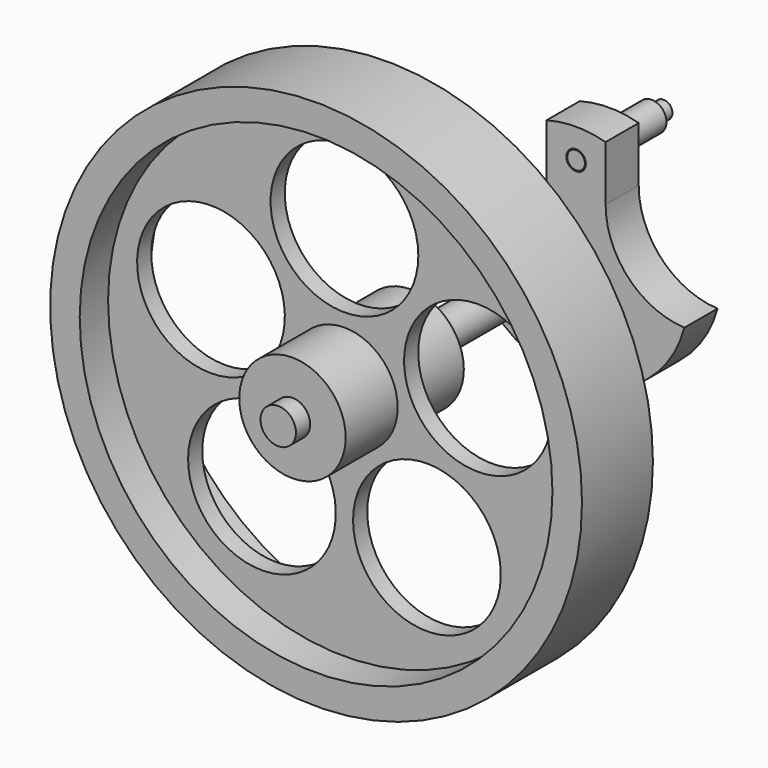
from build123d import *

# Parameters (mm, degrees)
F1_DEPTH         = 7
F2_D             = 6
F3_D             = 3.3
F4_R             = 2.5
F5_DEPTH         = 9
F6_R             = 2
F7_DEPTH         = 7
F8_R             = 1.5
F9_DEPTH         = 3
F10_SIZE         = 0.5
F11_R            = 3
F12_DEPTH        = 70
F16_D            = 6
F17_R            = 12.5
F18_DEPTH        = 68.001
F18_COPIES_COUNT = 5


# Not quite as in the source:
# - a pattern or mirror of a feature is missing from the dataset's text; its kind, count and spacing are read off the source's solid


with BuildPart() as f1:
    # F0 (on Front) → F1 (new body)
    with BuildSketch(Plane.XZ):
        with BuildLine():
            Line((5, 9), (5, 18.3303027798))
            ThreePointArc((5, 18.3303027798), (0, 19), (-5, 18.3303027798))
            Line((-5, 18.3303027798), (-5, 9))
            ThreePointArc((-5, 9), (-8.8679852531, -0.6613807072), (-18.3346110241, -4.9841788286))
            ThreePointArc((-18.3346110241, -4.9841788286), (0, -19), (18.3346110241, -4.9841788286))
            ThreePointArc((18.3346110241, -4.9841788286), (8.8679852531, -0.6613807072), (5, 9))
        make_face()
    extrude(amount=F1_DEPTH)

    # F2 (through all)
    with Locations(Plane(origin=(0, 0, 0), x_dir=(1, 0, 0), z_dir=(0, 1, 0))):
        with Locations((0, 0)):
            Hole(F2_D / 2)

    # F3 (through all)
    with Locations(Plane(origin=(0, 0, 0), x_dir=(1, 0, 0), z_dir=(0, 1, 0))):
        with Locations((0, -14)):
            Hole(F3_D / 2)


with BuildPart() as f5:
    # F4 (on face) → F5 (new body)
    with BuildSketch(Plane(origin=(0, 0, 0), x_dir=(-1, 0, 0), z_dir=(0, 1, 0))):
        with Locations((0, 14)):
            Circle(F4_R)
    extrude(amount=F5_DEPTH)

    # F6 (on face) → F7 (join)
    with BuildSketch(Plane.XZ):
        with Locations((0, 14)):
            Circle(F6_R)
    extrude(amount=F7_DEPTH)

    # F8 (on face) → F9 (join)
    with BuildSketch(Plane(origin=(0, 9, 0), x_dir=(-1, 0, 0), z_dir=(0, 1, 0))):
        with Locations((0, 14)):
            Circle(F8_R)
    extrude(amount=F9_DEPTH)

    # F10
    f10_edges = [f5.edges().sort_by_distance(p)[0] for p in [
        (1.5, 12, 14),
        (-2, -7, 14),
    ]]
    chamfer(f10_edges, length=F10_SIZE)


with BuildPart() as f12:
    # F11 (on Front) → F12 (new body)
    with BuildSketch(Plane.XZ):
        Circle(F11_R)
    extrude(amount=F12_DEPTH)


with BuildPart() as f14:
    # F13 (on Top) → F14 (revolve)
    with BuildSketch(Plane.XY):
        Polygon((0, -42), (0, -67), (9, -67), (9, -56), (40, -56), (40, -62), (45, -62), (45, -47), (40, -47), (40, -53), (9, -53), (9, -42), align=None)
    revolve(axis=Axis((0, -63.0867569871, 0), (0, -1, 0)))

    # F16 (through all)
    with Locations(Plane.XZ.offset(67)):
        with Locations((0, 0)):
            Hole(F16_D / 2)

    # F17 (on face) → F18 (cut, through all)
    with BuildSketch(Plane.XZ.offset(56)):
        with Locations((0, 23.75)):
            Circle(F17_R)
    f18 = extrude(amount=-F18_DEPTH, mode=Mode.SUBTRACT)

    # F18_copies: F18 ×5 about axis
    f18_copies_axis = Axis((0, 0, 0), (0, 1, 0))
    for i in range(1, F18_COPIES_COUNT):
        add(f18.rotate(f18_copies_axis, i * 360 / F18_COPIES_COUNT), mode=Mode.SUBTRACT)


solid = Compound([f1.part, f5.part, f12.part, f14.part])
